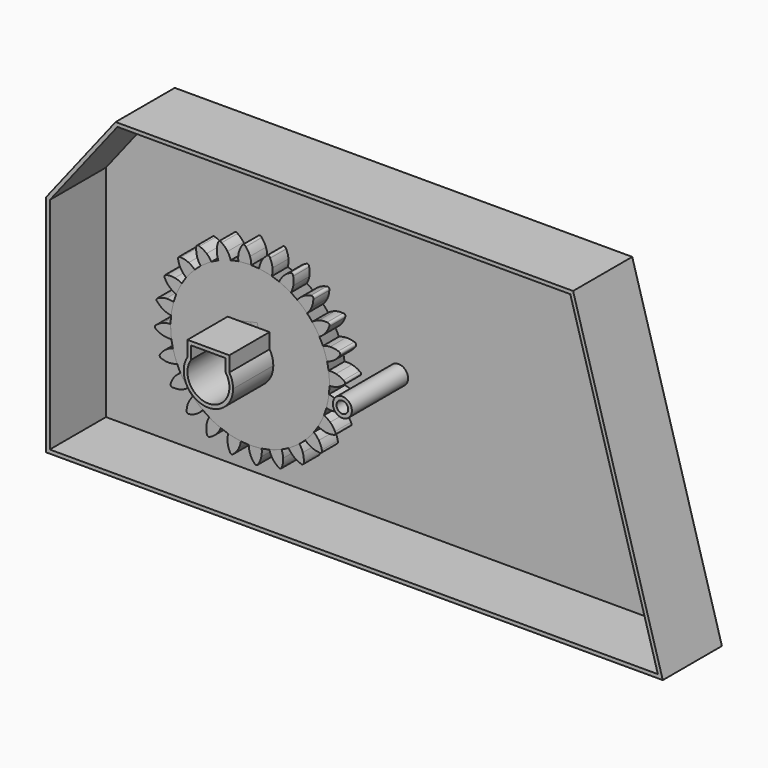
from build123d import *

# Parameters (mm, degrees)
F1_DEPTH = 16
F2_COUNT = 24
F3_R     = 3.9385625542
F4_DEPTH = 50
F5_T     = -2.5


with BuildPart() as f1:
    # F0 (on Front) → F1 (new body)
    with BuildSketch(Plane.XZ):
        with BuildLine():
            ThreePointArc((-7.8842675869, 53.139290225), (-3.5135215054, 53.6059792153), (0.8807473744, 53.7137796572))
            ThreePointArc((0.8807473744, 53.7137796572), (0.6461161172, 56.2304218962), (0, 58.674))
            ThreePointArc((0, 58.674), (-1.1904645717, 61.1974845451), (-2.8564405638, 63.4357213824))
            ThreePointArc((-2.8564405638, 63.4357213824), (-4.2119084037, 64.2613042219), (-5.448019844, 63.2658603022))
            ThreePointArc((-5.448019844, 63.2658603022), (-6.8075946488, 60.8293183888), (-7.6584938023, 58.1720357962))
            ThreePointArc((-7.6584938023, 58.1720357962), (-7.9801313613, 55.6650277654), (-7.8842675869, 53.139290225))
        make_face()
        with BuildLine():
            ThreePointArc((-7.8842675869, 53.139290225), (-35.0884247435, -40.6785974441), (53.721, 0))
            ThreePointArc((53.721, 0), (38.2966086664, 37.6738052983), (0.8807473744, 53.7137796572))
            ThreePointArc((0.8807473744, 53.7137796572), (-3.5135215054, 53.6059792153), (-7.8842675869, 53.139290225))
        make_face()
        with BuildLine():
            ThreePointArc((10.0692095664, 12.1012112428), (14.2852600623, 6.7767340583), (15.7888786842, 0.1537234052))
            ThreePointArc((15.7888786842, 0.1537234052), (-6.9508166509, -13.2802328295), (-7.7436098978, 13.1193202522))
            Line((-7.7436098978, 13.1193202522), (-7.7436098978, 19.4000941948))
            Line((-7.7436098978, 19.4000941948), (10.0692095664, 18.8254691035))
            Line((10.0692095664, 18.8254691035), (10.0692095664, 12.1012112428))
        make_face(mode=Mode.SUBTRACT)
    extrude(amount=F1_DEPTH)


with BuildPart() as f2_1:
    # F2: instance of F1
    add(f1.part.rotate(Axis((0, 0, 0), (0, 1, 0)), 1 * 360 / F2_COUNT))


with BuildPart() as f2_2:
    # F2: instance of F1
    add(f1.part.rotate(Axis((0, 0, 0), (0, 1, 0)), 2 * 360 / F2_COUNT))


with BuildPart() as f2_3:
    # F2: instance of F1
    add(f1.part.rotate(Axis((0, 0, 0), (0, 1, 0)), 3 * 360 / F2_COUNT))


with BuildPart() as f2_4:
    # F2: instance of F1
    add(f1.part.rotate(Axis((0, 0, 0), (0, 1, 0)), 4 * 360 / F2_COUNT))


with BuildPart() as f2_5:
    # F2: instance of F1
    add(f1.part.rotate(Axis((0, 0, 0), (0, 1, 0)), 5 * 360 / F2_COUNT))


with BuildPart() as f2_6:
    # F2: instance of F1
    add(f1.part.rotate(Axis((0, 0, 0), (0, 1, 0)), 6 * 360 / F2_COUNT))


with BuildPart() as f2_7:
    # F2: instance of F1
    add(f1.part.rotate(Axis((0, 0, 0), (0, 1, 0)), 7 * 360 / F2_COUNT))


with BuildPart() as f2_8:
    # F2: instance of F1
    add(f1.part.rotate(Axis((0, 0, 0), (0, 1, 0)), 8 * 360 / F2_COUNT))


with BuildPart() as f2_9:
    # F2: instance of F1
    add(f1.part.rotate(Axis((0, 0, 0), (0, 1, 0)), 9 * 360 / F2_COUNT))


with BuildPart() as f2_10:
    # F2: instance of F1
    add(f1.part.rotate(Axis((0, 0, 0), (0, 1, 0)), 10 * 360 / F2_COUNT))


with BuildPart() as f2_11:
    # F2: instance of F1
    add(f1.part.rotate(Axis((0, 0, 0), (0, 1, 0)), 11 * 360 / F2_COUNT))


with BuildPart() as f2_12:
    # F2: instance of F1
    add(f1.part.rotate(Axis((0, 0, 0), (0, 1, 0)), 12 * 360 / F2_COUNT))


with BuildPart() as f2_13:
    # F2: instance of F1
    add(f1.part.rotate(Axis((0, 0, 0), (0, 1, 0)), 13 * 360 / F2_COUNT))


with BuildPart() as f2_14:
    # F2: instance of F1
    add(f1.part.rotate(Axis((0, 0, 0), (0, 1, 0)), 14 * 360 / F2_COUNT))


with BuildPart() as f2_15:
    # F2: instance of F1
    add(f1.part.rotate(Axis((0, 0, 0), (0, 1, 0)), 15 * 360 / F2_COUNT))


with BuildPart() as f2_16:
    # F2: instance of F1
    add(f1.part.rotate(Axis((0, 0, 0), (0, 1, 0)), 16 * 360 / F2_COUNT))


with BuildPart() as f2_17:
    # F2: instance of F1
    add(f1.part.rotate(Axis((0, 0, 0), (0, 1, 0)), 17 * 360 / F2_COUNT))


with BuildPart() as f2_18:
    # F2: instance of F1
    add(f1.part.rotate(Axis((0, 0, 0), (0, 1, 0)), 18 * 360 / F2_COUNT))


with BuildPart() as f2_19:
    # F2: instance of F1
    add(f1.part.rotate(Axis((0, 0, 0), (0, 1, 0)), 19 * 360 / F2_COUNT))


with BuildPart() as f2_20:
    # F2: instance of F1
    add(f1.part.rotate(Axis((0, 0, 0), (0, 1, 0)), 20 * 360 / F2_COUNT))


with BuildPart() as f2_21:
    # F2: instance of F1
    add(f1.part.rotate(Axis((0, 0, 0), (0, 1, 0)), 21 * 360 / F2_COUNT))


with BuildPart() as f2_22:
    # F2: instance of F1
    add(f1.part.rotate(Axis((0, 0, 0), (0, 1, 0)), 22 * 360 / F2_COUNT))


with BuildPart() as f2_23:
    # F2: instance of F1
    add(f1.part.rotate(Axis((0, 0, 0), (0, 1, 0)), 23 * 360 / F2_COUNT))


with BuildPart() as f4:
    # F3 (on Front) → F4 (new body)
    with BuildSketch(Plane.XZ):
        Polygon((-63.6753439903, 131.7894458771), (-110.7138618827, 71.7433527191), (-110.7138618827, -80.1898017526), (306.3688576221, -80.1898017526), (245.7079440355, 131.7894458771), align=None)
        with BuildLine():
            ThreePointArc((10.7150094085, 6.889880588), (12.6143743289, 3.0256211841), (13.267535524, -1.2303708618))
            ThreePointArc((13.267535524, -1.2303708618), (-5.1497771024, -14.7795789773), (-12.6024631263, 6.836061563))
            Line((-12.6024631263, 6.836061563), (-12.6024631263, 15.3979491442))
            Line((-12.6024631263, 15.3979491442), (10.7150094085, 15.3979491442))
            Line((10.7150094085, 15.3979491442), (10.7150094085, 6.889880588))
        make_face(mode=Mode.SUBTRACT)
        with Locations((89.6744132042, 11.8231130764)):
            Circle(F3_R, mode=Mode.SUBTRACT)
    extrude(amount=F4_DEPTH)

    # F5
    f5_openings = [f4.faces().sort_by_distance(p)[0] for p in [
        (86.977321, -50, 21.670217),
    ]]
    offset(amount=F5_T, openings=f5_openings, kind=Kind.INTERSECTION)


solid = Compound([f1.part, f2_1.part, f2_2.part, f2_3.part, f2_4.part, f2_5.part, f2_6.part, f2_7.part, f2_8.part, f2_9.part, f2_10.part, f2_11.part, f2_12.part, f2_13.part, f2_14.part, f2_15.part, f2_16.part, f2_17.part, f2_18.part, f2_19.part, f2_20.part, f2_21.part, f2_22.part, f2_23.part, f4.part])
